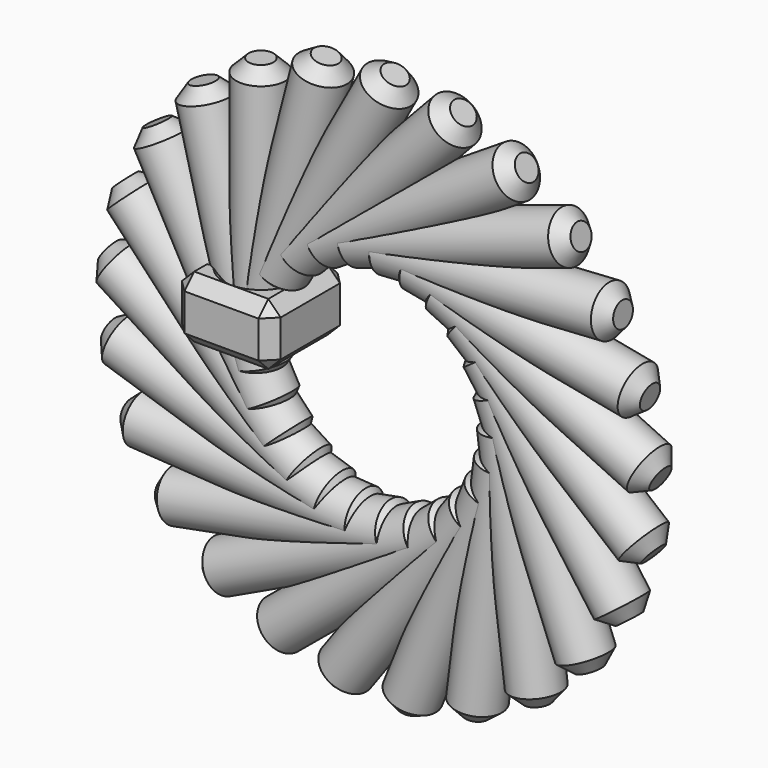
from build123d import *

# Parameters (mm, degrees)
F0_W      = 40
F0_H      = 40
F0_R      = 10
F1_DEPTH  = 25
F2_DEPTH  = 100
F3_SIZE   = 4.99999
F3_2_SIZE = 4.99999
F5_COUNT  = 25


# Not quite as in the source:
# - a fillet or chamfer is up to 0.001 mm smaller than in the source, because OpenCascade refuses the exact size


with BuildPart() as f1:
    # F0 (on Top) → F1 (new body)
    with BuildSketch(Plane.XY):
        Rectangle(F0_W, F0_H)
        Circle(F0_R, mode=Mode.SUBTRACT)
    extrude(amount=F1_DEPTH)

    # F3#2 (size 5 in the source; OpenCascade refuses exactly that, so slightly less here)
    f3_2_edges = [f1.edges().sort_by_distance(p)[0] for p in [
        (0, 20, 25),
        (20, 0, 25),
        (20, 20, 12.5),
        (-20, 20, 12.5),
        (0, 20, 0),
        (-20, -20, 12.5),
        (-20, 0, 0),
        (-20, 0, 25),
        (20, -20, 12.5),
        (0, -20, 0),
        (0, -20, 25),
        (20, 0, 0),
        (-10, 0, 0),
        (-10, 0, 25),
    ]]
    chamfer(f3_2_edges, length=F3_2_SIZE)


with BuildPart() as f2:
    # F0 (on Top) → F2 (new body)
    with BuildSketch(Plane.XY):
        Circle(F0_R)
    extrude(amount=F2_DEPTH)

    # F3 (size 5 in the source; OpenCascade refuses exactly that, so slightly less here)
    f3_edges = [f2.edges().sort_by_distance(p)[0] for p in [
        (-10, 0, 100),
        (-10, 0, 0),
    ]]
    chamfer(f3_edges, length=F3_SIZE)


with BuildPart() as f5_1:
    # F5: instance of F2
    add(f2.part.rotate(Axis((50, 0, 0), (0, -1, 0)), 1 * 360 / F5_COUNT))


with BuildPart() as f5_2:
    # F5: instance of F2
    add(f2.part.rotate(Axis((50, 0, 0), (0, -1, 0)), 2 * 360 / F5_COUNT))


with BuildPart() as f5_3:
    # F5: instance of F2
    add(f2.part.rotate(Axis((50, 0, 0), (0, -1, 0)), 3 * 360 / F5_COUNT))


with BuildPart() as f5_4:
    # F5: instance of F2
    add(f2.part.rotate(Axis((50, 0, 0), (0, -1, 0)), 4 * 360 / F5_COUNT))


with BuildPart() as f5_5:
    # F5: instance of F2
    add(f2.part.rotate(Axis((50, 0, 0), (0, -1, 0)), 5 * 360 / F5_COUNT))


with BuildPart() as f5_6:
    # F5: instance of F2
    add(f2.part.rotate(Axis((50, 0, 0), (0, -1, 0)), 6 * 360 / F5_COUNT))


with BuildPart() as f5_7:
    # F5: instance of F2
    add(f2.part.rotate(Axis((50, 0, 0), (0, -1, 0)), 7 * 360 / F5_COUNT))


with BuildPart() as f5_8:
    # F5: instance of F2
    add(f2.part.rotate(Axis((50, 0, 0), (0, -1, 0)), 8 * 360 / F5_COUNT))


with BuildPart() as f5_9:
    # F5: instance of F2
    add(f2.part.rotate(Axis((50, 0, 0), (0, -1, 0)), 9 * 360 / F5_COUNT))


with BuildPart() as f5_10:
    # F5: instance of F2
    add(f2.part.rotate(Axis((50, 0, 0), (0, -1, 0)), 10 * 360 / F5_COUNT))


with BuildPart() as f5_11:
    # F5: instance of F2
    add(f2.part.rotate(Axis((50, 0, 0), (0, -1, 0)), 11 * 360 / F5_COUNT))


with BuildPart() as f5_12:
    # F5: instance of F2
    add(f2.part.rotate(Axis((50, 0, 0), (0, -1, 0)), 12 * 360 / F5_COUNT))


with BuildPart() as f5_13:
    # F5: instance of F2
    add(f2.part.rotate(Axis((50, 0, 0), (0, -1, 0)), 13 * 360 / F5_COUNT))


with BuildPart() as f5_14:
    # F5: instance of F2
    add(f2.part.rotate(Axis((50, 0, 0), (0, -1, 0)), 14 * 360 / F5_COUNT))


with BuildPart() as f5_15:
    # F5: instance of F2
    add(f2.part.rotate(Axis((50, 0, 0), (0, -1, 0)), 15 * 360 / F5_COUNT))


with BuildPart() as f5_16:
    # F5: instance of F2
    add(f2.part.rotate(Axis((50, 0, 0), (0, -1, 0)), 16 * 360 / F5_COUNT))


with BuildPart() as f5_17:
    # F5: instance of F2
    add(f2.part.rotate(Axis((50, 0, 0), (0, -1, 0)), 17 * 360 / F5_COUNT))


with BuildPart() as f5_18:
    # F5: instance of F2
    add(f2.part.rotate(Axis((50, 0, 0), (0, -1, 0)), 18 * 360 / F5_COUNT))


with BuildPart() as f5_19:
    # F5: instance of F2
    add(f2.part.rotate(Axis((50, 0, 0), (0, -1, 0)), 19 * 360 / F5_COUNT))


with BuildPart() as f5_20:
    # F5: instance of F2
    add(f2.part.rotate(Axis((50, 0, 0), (0, -1, 0)), 20 * 360 / F5_COUNT))


with BuildPart() as f5_21:
    # F5: instance of F2
    add(f2.part.rotate(Axis((50, 0, 0), (0, -1, 0)), 21 * 360 / F5_COUNT))


with BuildPart() as f5_22:
    # F5: instance of F2
    add(f2.part.rotate(Axis((50, 0, 0), (0, -1, 0)), 22 * 360 / F5_COUNT))


with BuildPart() as f5_23:
    # F5: instance of F2
    add(f2.part.rotate(Axis((50, 0, 0), (0, -1, 0)), 23 * 360 / F5_COUNT))


with BuildPart() as f5_24:
    # F5: instance of F2
    add(f2.part.rotate(Axis((50, 0, 0), (0, -1, 0)), 24 * 360 / F5_COUNT))


solid = Compound([f1.part, f2.part, f5_1.part, f5_2.part, f5_3.part, f5_4.part, f5_5.part, f5_6.part, f5_7.part, f5_8.part, f5_9.part, f5_10.part, f5_11.part, f5_12.part, f5_13.part, f5_14.part, f5_15.part, f5_16.part, f5_17.part, f5_18.part, f5_19.part, f5_20.part, f5_21.part, f5_22.part, f5_23.part, f5_24.part])
